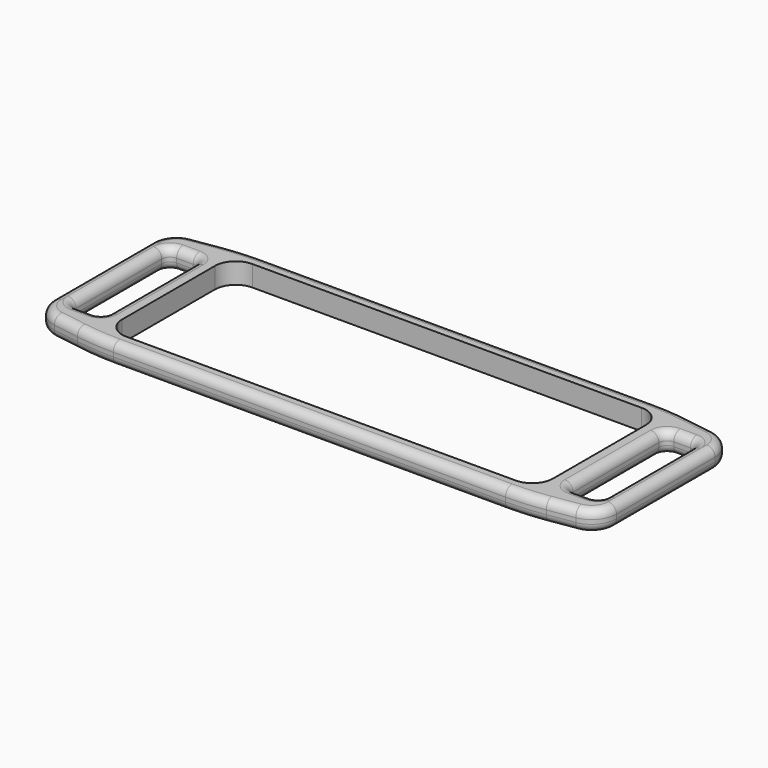
from build123d import *

# Parameters (mm, degrees)
F1_DEPTH = 2.5
F2_R     = 3
F3_R     = 30
F4_R     = 0.99999


# Not quite as in the source:
# - a fillet or chamfer is up to 0.001 mm smaller than in the source, because OpenCascade refuses the exact size


with BuildPart() as f1:
    # F0 (on Top) → F1 (new body)
    with BuildSketch(Plane.XY):
        Polygon((-26, -11.25), (26, -11.25), (34, -10), (34, 10), (26, 11.25), (-26, 11.25), (-34, 10), (-34, -10), align=None)
        with BuildLine():
            Line((-32, -6.46875), (-32, 6.46875))
            ThreePointArc((-32, 6.46875), (-31.7071067812, 7.1758567812), (-31, 7.46875))
            Line((-31, 7.46875), (-29, 7.46875))
            ThreePointArc((-29, 7.46875), (-28.2928932188, 7.1758567812), (-28, 6.46875))
            Line((-28, 6.46875), (-28, -6.46875))
            ThreePointArc((-28, -6.46875), (-28.2928932188, -7.1758567812), (-29, -7.46875))
            Line((-29, -7.46875), (-31, -7.46875))
            ThreePointArc((-31, -7.46875), (-31.7071067812, -7.1758567812), (-32, -6.46875))
        make_face(mode=Mode.SUBTRACT)
        with BuildLine():
            Line((-23.5, 9.5), (23.5, 9.5))
            ThreePointArc((23.5, 9.5), (25.267766953, 8.767766953), (26, 7))
            Line((26, 7), (26, -7))
            ThreePointArc((26, -7), (25.267766953, -8.767766953), (23.5, -9.5))
            Line((23.5, -9.5), (-23.5, -9.5))
            ThreePointArc((-23.5, -9.5), (-25.267766953, -8.767766953), (-26, -7))
            Line((-26, -7), (-26, 7))
            ThreePointArc((-26, 7), (-25.267766953, 8.767766953), (-23.5, 9.5))
        make_face(mode=Mode.SUBTRACT)
        with BuildLine():
            ThreePointArc((32, -6.46875), (31.7071067812, -7.1758567812), (31, -7.46875))
            Line((31, -7.46875), (29, -7.46875))
            ThreePointArc((29, -7.46875), (28.2928932188, -7.1758567812), (28, -6.46875))
            Line((28, -6.46875), (28, 6.46875))
            ThreePointArc((28, 6.46875), (28.2928932188, 7.1758567812), (29, 7.46875))
            Line((29, 7.46875), (31, 7.46875))
            ThreePointArc((31, 7.46875), (31.7071067812, 7.1758567812), (32, 6.46875))
            Line((32, 6.46875), (32, -6.46875))
        make_face(mode=Mode.SUBTRACT)
    extrude(amount=F1_DEPTH)

    # F2
    f2_edges = [f1.edges().sort_by_distance(p)[0] for p in [
        (34, -10, 1.25),
        (34, 10, 1.25),
        (-34, -10, 1.25),
        (-34, 10, 1.25),
    ]]
    fillet(f2_edges, radius=F2_R)

    # F3
    f3_edges = [f1.edges().sort_by_distance(p)[0] for p in [
        (-26, -11.25, 1.25),
        (26, -11.25, 1.25),
        (-26, 11.25, 1.25),
        (26, 11.25, 1.25),
    ]]
    fillet(f3_edges, radius=F3_R)

    # F4 (radius 1 in the source; OpenCascade refuses exactly that, so slightly less here)
    f4_edges = [f1.edges().sort_by_distance(p)[0] for p in [
        (0, -11.25, 2.5),
        (28, 0, 2.5),
        (-32, 0, 2.5),
        (-30, 7.46875, 0),
        (30, 7.46875, 0),
        (33.279188, -9.383069, 0),
    ]]
    fillet(f4_edges, radius=F4_R)


solid = f1.part
